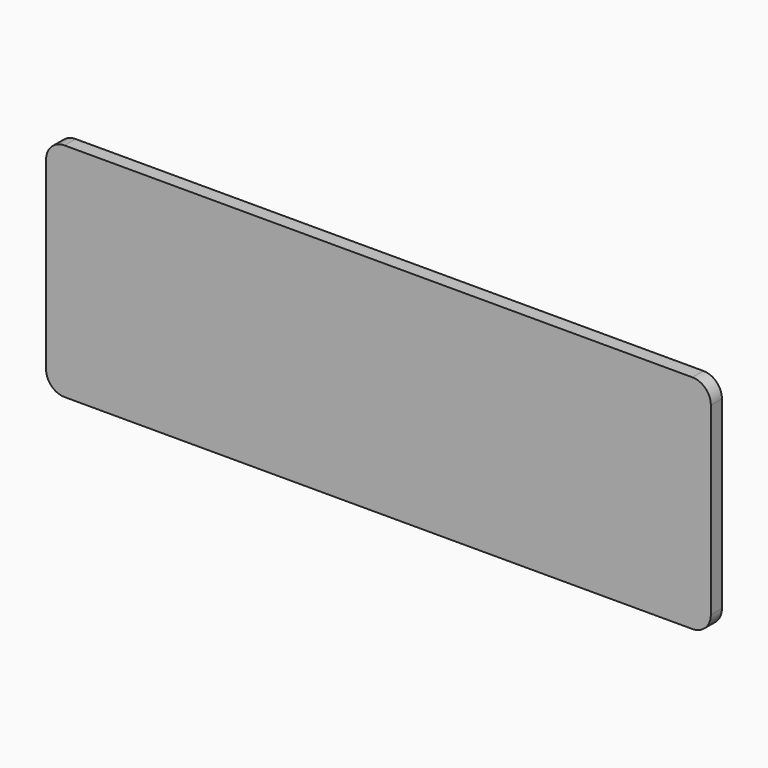
from build123d import *

# Parameters (mm, degrees)
F1_DEPTH = 19.05
F3_DEPTH = 9.525
F4_R     = 25.4
F5_R     = 25.4
F6_R     = 25.4
F7_R     = 25.4


# Not quite as in the source:
# - a length typed as a fraction of an inch, garbled in the dataset ("3 / 203.2 mm" for 3/8 in), is restored


with BuildPart() as f1:
    # F0 (on Front) → F1 (new body)
    with BuildSketch(Plane.XZ):
        Polygon((457.2, 163.4292998382), (0, 163.4292998382), (-457.2, 163.4292998382), (-457.2, -141.3707001618), (0, -141.3707001618), (457.2, -141.3707001618), align=None)
    extrude(amount=F1_DEPTH)

    # F2 (on Front) → F3 (cut)
    with BuildSketch(Plane.XZ):
        Polygon((425.45, -106.4507083202), (425.45, 13.6912916798), (425.45, 133.8332916798), (406.4, 133.8332916798), (406.4, 23.3432916798), (406.4, 13.6912916798), (406.4, 4.0392916798), (406.4, -106.4507083202), align=None)
        Polygon((406.4, 13.6912916798), (406.4, 23.3432916798), (-406.4, 23.3432916798), (-406.4, 13.6912916798), (-406.4, 4.0392916798), (406.4, 4.0392916798), align=None)
        Polygon((-406.4, 13.6912916798), (-406.4, 23.3432916798), (-406.4, 133.8332916798), (-425.45, 133.8332916798), (-425.45, 13.6912916798), (-425.45, -106.4507083202), (-406.4, -106.4507083202), (-406.4, 4.0392916798), align=None)
    extrude(amount=F3_DEPTH, mode=Mode.SUBTRACT)

    # F4
    f4_edges = [f1.edges().sort_by_distance(p)[0] for p in [
        (457.2, -9.525, 163.4293),
    ]]
    fillet(f4_edges, radius=F4_R)

    # F5
    f5_edges = [f1.edges().sort_by_distance(p)[0] for p in [
        (457.2, -9.525, -141.3707),
    ]]
    fillet(f5_edges, radius=F5_R)

    # F6
    f6_edges = [f1.edges().sort_by_distance(p)[0] for p in [
        (-457.2, -9.525, 163.4293),
    ]]
    fillet(f6_edges, radius=F6_R)

    # F7
    f7_edges = [f1.edges().sort_by_distance(p)[0] for p in [
        (-457.2, -9.525, -141.3707),
    ]]
    fillet(f7_edges, radius=F7_R)


solid = f1.part
